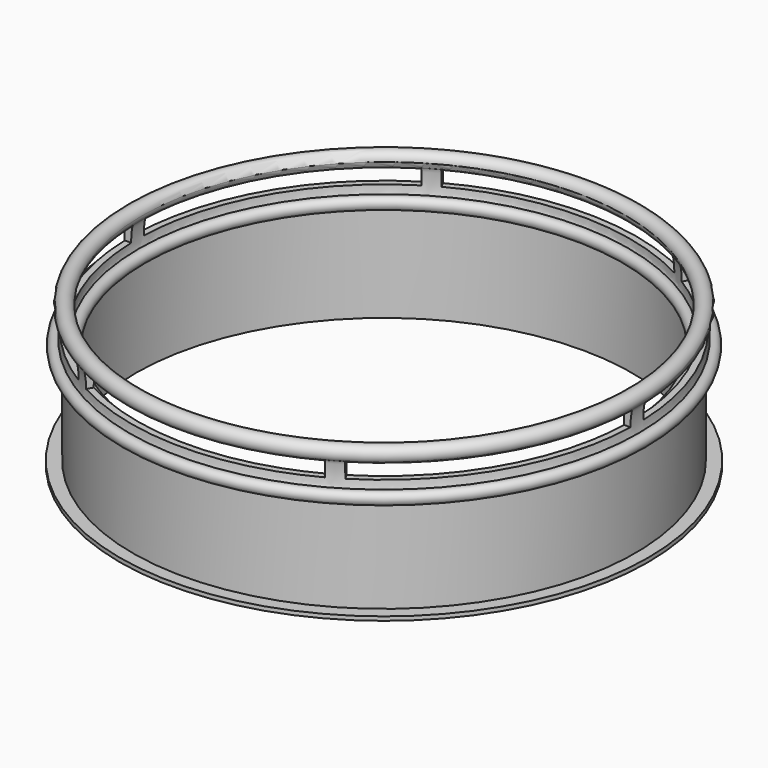
from build123d import *

# Parameters (mm, degrees)
F6_DEPTH = 25.4


with BuildPart() as f3:
    # F0 (on Front) → F3 (revolve)
    with BuildSketch(Plane.XZ):
        with BuildLine():
            ThreePointArc((8.5900427721, -9.3542057479), (11.6271996458, -5.10864252), (12.7, 0))
            ThreePointArc((12.7, 0), (-5.10864252, 11.6271996458), (-8.5900427721, -9.3542057479))
            ThreePointArc((-8.5900427721, -9.3542057479), (0, -12.7), (8.5900427721, -9.3542057479))
        make_face()
        with BuildLine():
            ThreePointArc((8.5900427721, -9.3542057479), (0, -12.7), (-8.5900427721, -9.3542057479))
            add(Edge.make_bspline(
                [(-12.7, -50.8), (-11.3931018859, -52.2795841098), (-9.3920831721, -53.014888066), (-3.7697998276, -47.9313603441), (-5.0543149936, -12.8899302213), (-8.5900427721, -9.3542057479)],
                knots=[0, 0, 0, 0, 0.1767774153, 0.4153705122, 1, 1, 1, 1], degree=3))
            ThreePointArc((-12.7, -50.8), (-19.05, -57.15), (-12.7, -63.5))
            Line((-12.7, -63.5), (0, -63.5))
            Line((0, -63.5), (12.7, -63.5))
            ThreePointArc((12.7, -63.5), (19.05, -57.15), (12.7, -50.8))
            add(Edge.make_bspline(
                [(12.7, -50.8), (11.3931018859, -52.2795841098), (9.3920831721, -53.014888066), (3.7697998276, -47.9313603441), (5.0543149936, -12.8899302213), (8.5900427721, -9.3542057479)],
                knots=[0, 0, 0, 0, 0.1767774153, 0.4153705122, 1, 1, 1, 1], degree=3))
        make_face()
    revolve(axis=Axis((400, 0, 1.716285944), (0, 0, -1)))

    # F5 (on offset) → F6 (cut)
    with BuildSketch(Plane.XY.offset(-10.16)):
        with BuildLine():
            Line((169.1226982685, -374.4912169133), (378.0029547439, -12.7))
            Line((378.0029547439, -12.7), (-39.7575582068, -12.7))
            ThreePointArc((-39.7575582068, -12.7), (19, -219.9704525612), (169.1226982685, -374.4912169133))
        make_face()
        with BuildLine():
            Line((-39.7575582068, 12.7), (378.0029547439, 12.7))
            Line((378.0029547439, 12.7), (169.1226982685, 374.4912169133))
            ThreePointArc((169.1226982685, 374.4912169133), (19, 219.9704525612), (-39.7575582068, 12.7))
        make_face()
        with BuildLine():
            Line((191.1197435247, 387.1912169133), (400, 25.4))
            Line((400, 25.4), (608.8802564753, 387.1912169133))
            ThreePointArc((608.8802564753, 387.1912169133), (400, 439.9409051225), (191.1197435247, 387.1912169133))
        make_face()
        with BuildLine():
            Line((630.8773017315, 374.4912169133), (421.9970452561, 12.7))
            Line((421.9970452561, 12.7), (839.7575582068, 12.7))
            ThreePointArc((839.7575582068, 12.7), (781, 219.9704525612), (630.8773017315, 374.4912169133))
        make_face()
        with BuildLine():
            Line((839.7575582068, -12.7), (421.9970452561, -12.7))
            Line((421.9970452561, -12.7), (630.8773017315, -374.4912169133))
            ThreePointArc((630.8773017315, -374.4912169133), (781, -219.9704525612), (839.7575582068, -12.7))
        make_face()
        with BuildLine():
            Line((608.8802564753, -387.1912169133), (400, -25.4))
            Line((400, -25.4), (191.1197435247, -387.1912169133))
            ThreePointArc((191.1197435247, -387.1912169133), (400, -439.9409051225), (608.8802564753, -387.1912169133))
        make_face()
    extrude(amount=-F6_DEPTH, mode=Mode.SUBTRACT)


with BuildPart() as f3b:
    # F0 (on Front) → F3, piece 2 (revolve)
    with BuildSketch(Plane.XZ):
        with BuildLine():
            add(Edge.make_bspline(
                [(-12.5602874905, -50.4275076091), (-13.3057196509, -50.4217364884), (-15.0249900236, -50.5822224615), (-19.2955921093, -53.1510410325), (-19.9441064961, -59.7254744963), (-15.902495506, -63.4365990904), (-14.2082123321, -63.7347346363), (-13.0495252088, -63.8175)],
                knots=[0, 0, 0, 0, 0.1539184024, 0.3669024694, 0.6101320409, 0.8303696922, 1, 1, 1, 1], degree=3))
            add(Edge.make_bspline(
                [(-12.5602874905, -50.4275076091), (-11.6419888001, -51.3184421844), (-9.698402422, -53.2045627617), (-6.5034250729, -48.7931724826), (-8.8975047251, -47.1046195233), (-16.423225527, -46.6603431424), (-22.1527686106, -53.459599144), (-21.2763745442, -60.5451581586), (-18.6975576855, -64.5279023886), (-16.3640286773, -66.1001577973), (-13.9314141124, -66.3575)],
                knots=[0, 0, 0, 0, 0.1025655414, 0.2132773125, 0.2943103446, 0.4443923591, 0.6057553629, 0.7524937718, 0.8711400896, 1, 1, 1, 1], degree=3))
            Line((-13.9314141124, -66.3575), (-2.54, -66.3575))
            Line((-2.54, -66.3575), (-2.54, -218.7575))
            Line((-2.54, -218.7575), (-22.86, -218.7575))
            Line((-22.86, -218.7575), (-22.86, -225.1075))
            Line((-22.86, -225.1075), (2.54, -225.1075))
            Line((2.54, -225.1075), (2.54, -218.7575))
            Line((2.54, -218.7575), (2.54, -66.3575))
            Line((2.54, -66.3575), (13.9314141124, -66.3575))
            add(Edge.make_bspline(
                [(12.5602874905, -50.4275076091), (11.6419888001, -51.3184421844), (9.698402422, -53.2045627617), (6.5034250729, -48.7931724826), (8.8975047251, -47.1046195233), (16.423225527, -46.6603431424), (22.1527686106, -53.459599144), (21.2763745442, -60.5451581586), (18.6975576855, -64.5279023886), (16.3640286773, -66.1001577973), (13.9314141124, -66.3575)],
                knots=[0, 0, 0, 0, 0.1025655414, 0.2132773125, 0.2943103446, 0.4443923591, 0.6057553629, 0.7524937718, 0.8711400896, 1, 1, 1, 1], degree=3))
            add(Edge.make_bspline(
                [(12.5602874905, -50.4275076091), (13.3057196509, -50.4217364884), (15.0249900236, -50.5822224615), (19.2955921093, -53.1510410325), (19.9441064961, -59.7254744963), (15.902495506, -63.4365990904), (14.2082123321, -63.7347346363), (13.0495252088, -63.8175)],
                knots=[0, 0, 0, 0, 0.1539184024, 0.3669024694, 0.6101320409, 0.8303696922, 1, 1, 1, 1], degree=3))
            Line((13.0495252088, -63.8175), (0, -63.8175))
            Line((0, -63.8175), (-13.0495252088, -63.8175))
        make_face()
    revolve(axis=Axis((400, 0, 1.716285944), (0, 0, -1)))


solid = Compound([f3.part, f3b.part])
